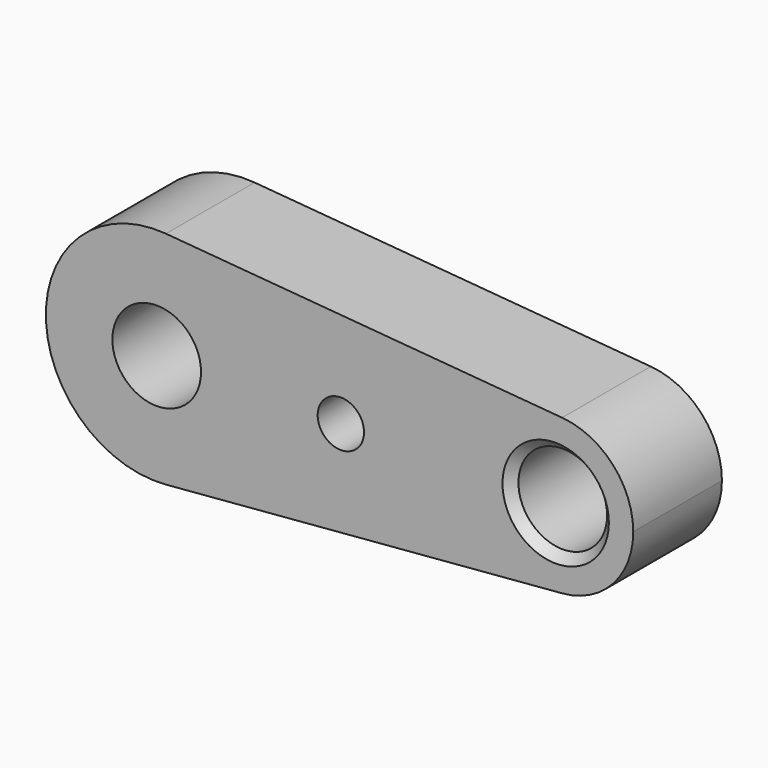
from build123d import *

# Parameters (mm, degrees)
F0_R     = 10
F1_DEPTH = 25
F2_SIZE  = 2
F6_R     = 5.2276340185
F7_DEPTH = 25


# Not quite as in the source:
# - the program builds the solid bodies; features that only make, move or delete a surface that nothing else refers to are left out


with BuildPart() as f1:
    # F0 (on Front) → F1 (new body)
    with BuildSketch(Plane.XZ):
        with BuildLine():
            ThreePointArc((2.0833333333, -24.9130432148), (18.3995018048, -16.9250800097), (25, 0))
            ThreePointArc((25, 0), (18.3995018048, 16.9250800097), (2.0833333333, 24.9130432148))
            ThreePointArc((2.0833333333, 24.9130432148), (-25, 0), (2.0833333333, -24.9130432148))
        make_face()
        Circle(F0_R, mode=Mode.SUBTRACT)
        with BuildLine():
            ThreePointArc((2.0833333333, 24.9130432148), (18.3995018048, 16.9250800097), (25, 0))
            ThreePointArc((25, 0), (18.3995018048, -16.9250800097), (2.0833333333, -24.9130432148))
            Line((2.0833333333, -24.9130432148), (91.4583333333, -17.4391302504))
            ThreePointArc((91.4583333333, -17.4391302504), (72.5, 0), (91.4583333333, 17.4391302504))
            Line((91.4583333333, 17.4391302504), (2.0833333333, 24.9130432148))
        make_face()
        with BuildLine():
            ThreePointArc((107.5, 0), (102.8796512634, 11.8475560068), (91.4583333333, 17.4391302504))
            ThreePointArc((91.4583333333, 17.4391302504), (72.5, 0), (91.4583333333, -17.4391302504))
            ThreePointArc((91.4583333333, -17.4391302504), (102.8796512634, -11.8475560068), (107.5, 0))
        make_face()
        with Locations((90, 0)):
            Circle(F0_R, mode=Mode.SUBTRACT)
    extrude(amount=F1_DEPTH)

    # F2
    f2_edges = [f1.edges().sort_by_distance(p)[0] for p in [
        (80, -25, 0),
    ]]
    chamfer(f2_edges, length=F2_SIZE)

    # F6 (on face) → F7 (cut)
    with BuildSketch(Plane.XZ.offset(25)):
        with Locations((41.5417253971, 0)):
            Circle(F6_R)
    extrude(amount=-F7_DEPTH, mode=Mode.SUBTRACT)


solid = f1.part
